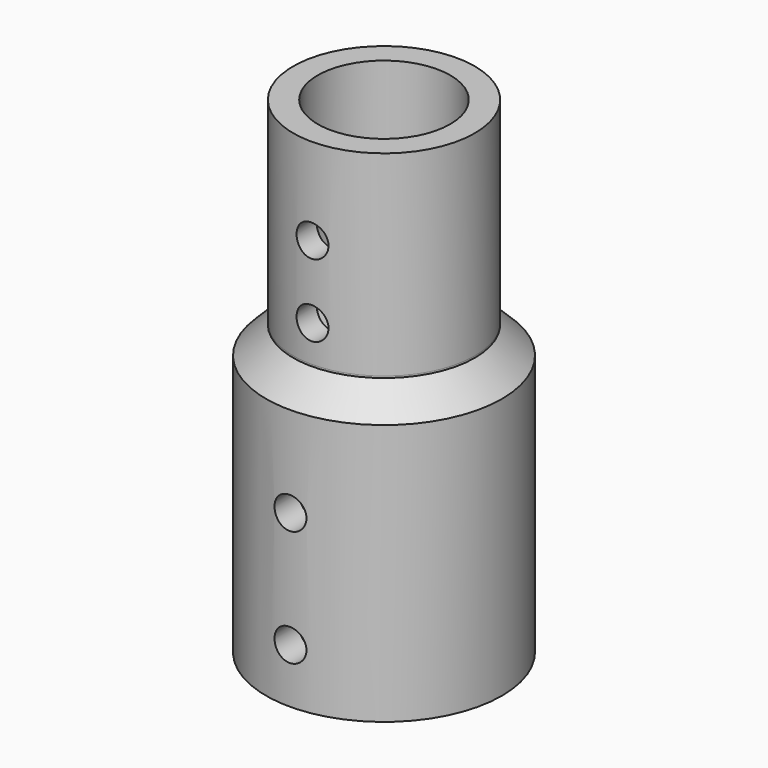
from build123d import *

# Parameters (mm, degrees)
F0_R        = 25
F0_R_2      = 18.25
F1_DEPTH    = 54
F4_D        = 8.8
F4_DEPTH    = 15.75
F4_START    = 1.3902459
F4_TIP      = 2.6437867237
F5_R        = 32.5
F6_DEPTH    = 80
F7_R        = 24.25
F8_DEPTH    = 70
F9_S5_R     = 25
F9_T6_DEPTH = 48
F12_D       = 8.8


# Not quite as in the source:
# - a fillet or chamfer that OpenCascade refuses, or shapes differently, is made with other operations: its cross-section is extruded or revolved along the edge and cut away or added


with BuildPart() as f1:
    # F0 (on Top) → F1 (new body)
    with BuildSketch(Plane.XY):
        Circle(F0_R)
        Circle(F0_R_2, mode=Mode.SUBTRACT)
    extrude(amount=F1_DEPTH)

    # F4
    # its depths count from where the whole tool has entered the part; down to there all is cleared
    with Locations(Plane.XZ.offset(26).offset(-F4_START)):
        with Locations((0, 10), (0, 30)):
            Hole(F4_D / 2, depth=F4_DEPTH)
            with Locations((0, 0, -(F4_DEPTH + F4_TIP / 2))):  # 118° drill point
                Cone(0, F4_D / 2, F4_TIP, mode=Mode.SUBTRACT)

    # F5 (on face) → F6 (join)
    with BuildSketch(Plane.XY):
        Circle(F5_R)
    extrude(amount=-F6_DEPTH)

    # F7 (on face) → F8 (cut)
    with BuildSketch(Plane(origin=(0, 0, -80), x_dir=(1, 0, 0), z_dir=(0, 0, -1))):
        Circle(F7_R)
    extrude(amount=-F8_DEPTH, mode=Mode.SUBTRACT)

    # F9: chamfer of 8 on 1 edges, made by hand


with BuildPart() as f9_tool2:
    # F9_s3 → F9_t4 (revolve)
    with BuildSketch(Plane.XZ):
        Polygon((32.5, -8), (24.5, 0), (32.5, 0), align=None)
    revolve(axis=Axis((0, 0, 0), (0, 0, 1)))

    # F9_s5 → F9_t6 (cut, symmetric)
    with BuildSketch(Plane.XY.offset(-4)):
        Circle(F9_S5_R)
    extrude(amount=F9_T6_DEPTH, both=True, mode=Mode.SUBTRACT)


with BuildPart() as f1_1:
    add(f1.part)

    # F9_t1: cut F9_tool2
    add(f9_tool2.part, mode=Mode.SUBTRACT)

    # F12 (through all)
    with Locations(Plane.XZ.offset(51)):
        with Locations((0, -33), (0, -65)):
            Hole(F12_D / 2)


solid = f1_1.part
